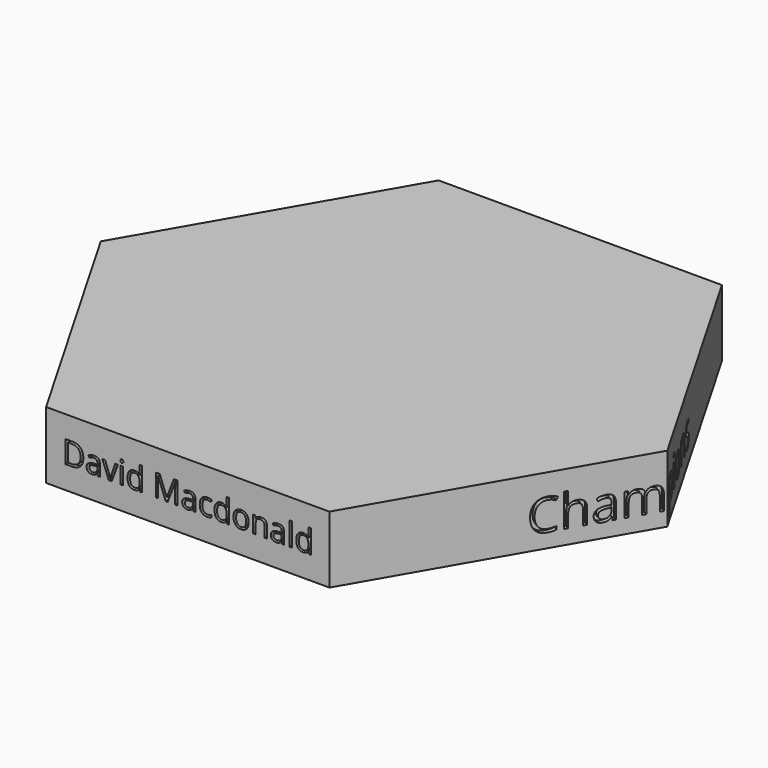
from build123d import *

# Parameters (mm, degrees)
F1_DEPTH      = 15
F2_TEXT_SIZE  = 6.9444444444
F3_DEPTH      = 1
F4_TEXT_SIZE  = 7.2036171332
F5_DEPTH      = 1
F6_TEXT_SIZE  = 9.6247408591
F7_DEPTH      = 1
F8_TEXT_SIZE  = 9.3021378335
F9_DEPTH      = 1
F10_TEXT_SIZE = 9.7222222222
F11_DEPTH     = 1
F12_TEXT_SIZE = 9.7222222222
F13_DEPTH     = 1


# Not quite as in the source:
# - Text() gives the source's letters only with a copy of the font that has no kerning and outlines rounded to 1/6400 em; it was checked with that copy


with BuildPart() as f1:
    # F0 (on Top) → F1 (new body)
    with BuildSketch(Plane.XY):
        Polygon((31.7542648054, 55), (-31.7542648054, 55), (-63.5085296109, 0), (-31.7542648054, -55), (31.7542648054, -55), (63.5085296109, 0), align=None)
    extrude(amount=F1_DEPTH)

    # F2 (on face) → F3 (cut)
    with BuildSketch(Plane.XZ.offset(55)):
        with Locations((-28.0490451389, 5.1254145169)):
            Text('David Macdonald', F2_TEXT_SIZE, font='Open Sans', text_align=(TextAlign.LEFT, TextAlign.BOTTOM))
    extrude(amount=-F3_DEPTH, mode=Mode.SUBTRACT)

    # F4 (on face) → F5 (cut)
    with BuildSketch(Plane(origin=(0, 55, 0), x_dir=(-1, 0, 0), z_dir=(0, 1, 0))):
        with Locations((-26.7850745186, 4.9382071011)):
            Text('Louis-Alexis A-D', F4_TEXT_SIZE, font='Open Sans', text_align=(TextAlign.LEFT, TextAlign.BOTTOM))
    extrude(amount=-F5_DEPTH, mode=Mode.SUBTRACT)

    # F6 (on face) → F7 (cut)
    with BuildSketch(Plane(origin=(-47.6313972081, 27.5, 0), x_dir=(-0.5, -0.8660254038, 0), z_dir=(-0.8660254038, 0.5, 0))):
        with Locations((20.6031002007, 3.9927139878)):
            Text('20', F6_TEXT_SIZE, font='Open Sans', text_align=(TextAlign.LEFT, TextAlign.BOTTOM))
    extrude(amount=-F7_DEPTH, mode=Mode.SUBTRACT)

    # F8 (on face) → F9 (cut)
    with BuildSketch(Plane(origin=(-47.6313972081, -27.5, 0), x_dir=(0.5, -0.8660254038, 0), z_dir=(-0.8660254038, -0.5, 0))):
        with Locations((-31.3925594091, 3.9951244835)):
            Text('17', F8_TEXT_SIZE, font='Open Sans', text_align=(TextAlign.LEFT, TextAlign.BOTTOM))
    extrude(amount=-F9_DEPTH, mode=Mode.SUBTRACT)

    # F10 (on face) → F11 (cut)
    with BuildSketch(Plane(origin=(47.6313972081, -27.5, 0), x_dir=(0.5, 0.8660254038, 0), z_dir=(0.8660254038, -0.5, 0))):
        with Locations((5.3614696665, 3.1997896731)):
            Text('Cham', F10_TEXT_SIZE, font='Open Sans', text_align=(TextAlign.LEFT, TextAlign.BOTTOM))
    extrude(amount=-F11_DEPTH, mode=Mode.SUBTRACT)

    # F12 (on face) → F13 (cut)
    with BuildSketch(Plane(origin=(47.6313972081, 27.5, 0), x_dir=(-0.5, 0.8660254038, 0), z_dir=(0.8660254038, 0.5, 0))):
        with Locations((-31.0861473381, 3.478960832)):
            Text('pions', F12_TEXT_SIZE, font='Open Sans', text_align=(TextAlign.LEFT, TextAlign.BOTTOM))
    extrude(amount=-F13_DEPTH, mode=Mode.SUBTRACT)


solid = f1.part
